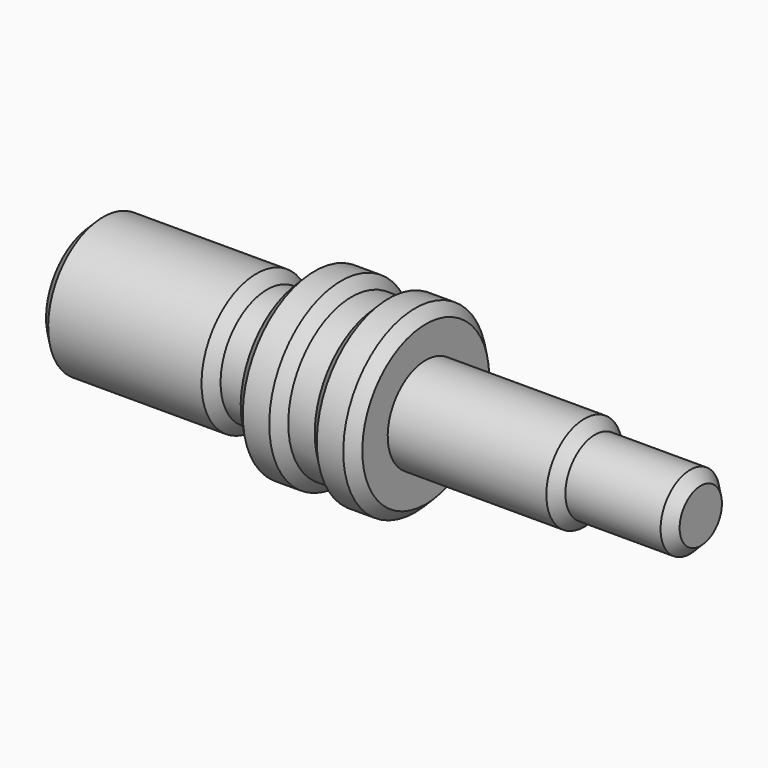
from build123d import *

# Parameters (mm, degrees)
F0_W    = 7
F0_H    = 11
F0_W_2  = 5
F0_H_2  = 15
F0_W_3  = 20
F0_H_3  = 7
F2_SIZE = 1.99999


# Not quite as in the source:
# - a fillet or chamfer is up to 0.001 mm smaller than in the source, because OpenCascade refuses the exact size


with BuildPart() as f1:
    # F0 (on Front) → F1 (revolve)
    with BuildSketch(Plane.XZ):
        Polygon((33, 0), (0, 0), (0, -13), (33, -13), (33, -11), align=None)
        with Locations((36.5, -5.5)):
            Rectangle(F0_W, F0_H)
        Polygon((49, 0), (40, 0), (40, -11), (40, -17), (49, -17), (49, -15), align=None)
        with Locations((51.5, -7.5)):
            Rectangle(F0_W_2, F0_H_2)
        Polygon((63, 0), (54, 0), (54, -15), (54, -17), (63, -17), (63, -9), align=None)
        Polygon((95, 0), (63, 0), (63, -9), (95, -9), (95, -7), align=None)
        with Locations((105, -3.5)):
            Rectangle(F0_W_3, F0_H_3)
    revolve(axis=Axis((51.5, 0, 0), (1, 0, 0)))

    # F2 (size 2 in the source; OpenCascade refuses exactly that, so slightly less here)
    f2_edges = [f1.edges().sort_by_distance(p)[0] for p in [
        (0, 0, 13),
        (33, 0, 13),
        (16.5, 0, -13),
        (40, 0, 17),
        (49, 0, 17),
        (54, 0, 17),
        (63, 0, 17),
        (95, 0, 9),
        (115, 0, 7),
    ]]
    chamfer(f2_edges, length=F2_SIZE)


solid = f1.part
